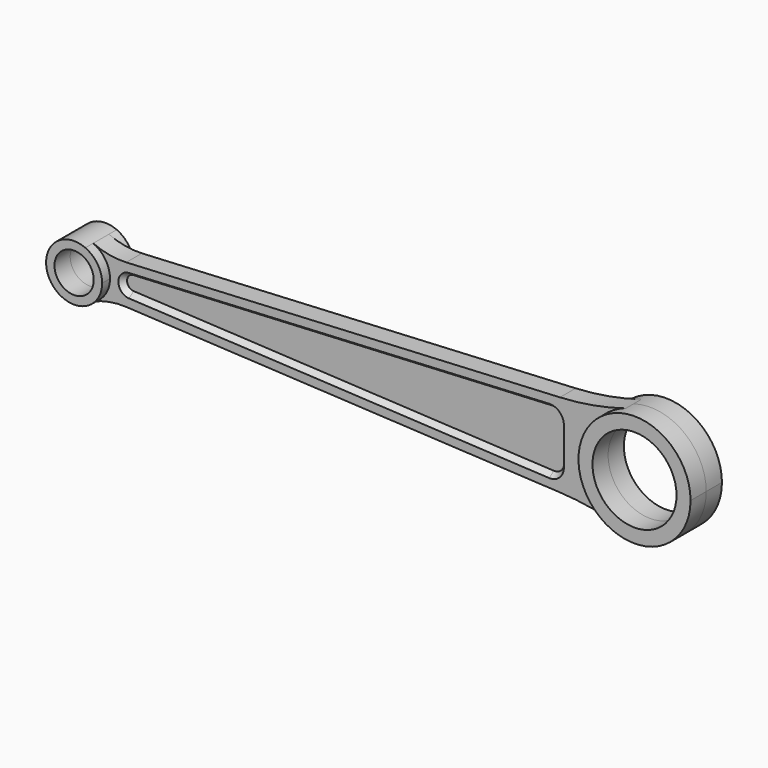
from build123d import *

# Parameters (mm, degrees)
F2_DEPTH = 3.5
F0_R     = 15
F0_R_2   = 7
F3_DEPTH = 7


# Not quite as in the source:
# - a pattern or mirror of a feature is missing from the dataset's text; its kind, count and spacing are read off the source's solid


with BuildPart() as f2:
    # F0 (on Front) → F2 (new body, symmetric)
    with BuildSketch(Plane.XZ):
        with BuildLine():
            ThreePointArc((4.0181641166, 9.157202473), (8.372026074, 5.4689285438), (10, 0))
            ThreePointArc((10, 0), (8.372026074, -5.4689285438), (4.0181641166, -9.157202473))
            ThreePointArc((4.0181641166, -9.157202473), (9.7812118117, -7.3913621026), (15.7960057944, -7))
            Line((15.7960057944, -7), (170.5928896385, -14.9325123484))
            ThreePointArc((170.5928896385, -14.9325123484), (182.467918995, -16.2860219438), (194.0827327125, -19.1046054094))
            ThreePointArc((194.0827327125, -19.1046054094), (180, 0), (194.0827327125, 19.1046054094))
            ThreePointArc((194.0827327125, 19.1046054094), (182.467918995, 16.2860219438), (170.5928896385, 14.9325123484))
            Line((170.5928896385, 14.9325123484), (15.7960057944, 7))
            ThreePointArc((15.7960057944, 7), (9.7812118117, 7.3913621026), (4.0181641166, 9.157202473))
        make_face()
    extrude(amount=F2_DEPTH, both=True)

    # F0 (on Front) → F3 (join, symmetric)
    with BuildSketch(Plane.XZ):
        with BuildLine():
            ThreePointArc((220, 0), (211.86706902, 16.0988407308), (194.0827327125, 19.1046054094))
            ThreePointArc((194.0827327125, 19.1046054094), (180, 0), (194.0827327125, -19.1046054094))
            ThreePointArc((194.0827327125, -19.1046054094), (211.86706902, -16.0988407308), (220, 0))
        make_face()
        with Locations((200, 0)):
            Circle(F0_R, mode=Mode.SUBTRACT)
        with BuildLine():
            ThreePointArc((4.0181641166, -9.157202473), (8.372026074, -5.4689285438), (10, 0))
            ThreePointArc((10, 0), (8.372026074, 5.4689285438), (4.0181641166, 9.157202473))
            ThreePointArc((4.0181641166, 9.157202473), (-10, 0), (4.0181641166, -9.157202473))
        make_face()
        Circle(F0_R_2, mode=Mode.SUBTRACT)
    extrude(amount=F3_DEPTH, both=True)

    # F5 (on offset) → F6 section 0
    with BuildSketch(Plane.XZ.offset(1.5)):
        with BuildLine():
            Line((166.8208787534, 10.1807990679), (16.8720562524, 2.496723933))
            ThreePointArc((16.8720562524, 2.496723933), (14.5, 0), (16.8720562524, -2.496723933))
            Line((16.8720562524, -2.496723933), (166.8208787534, -10.1807990679))
            ThreePointArc((166.8208787534, -10.1807990679), (169.4107131348, -9.2227980591), (170.5, -6.6853855618))
            Line((170.5, -6.6853855618), (170.5, 6.6853855618))
            ThreePointArc((170.5, 6.6853855618), (169.4107131348, 9.2227980591), (166.8208787534, 10.1807990679))
        make_face()
    # F4 (on face) → F6 section 1
    with BuildSketch(Plane.XZ.offset(3.5)):
        with BuildLine():
            Line((166.7441125049, 11.6788334277), (16.7952900039, 3.9947582928))
            ThreePointArc((16.7952900039, 3.9947582928), (13, 0), (16.7952900039, -3.9947582928))
            Line((16.7952900039, -3.9947582928), (166.7441125049, -11.6788334277))
            ThreePointArc((166.7441125049, -11.6788334277), (170.4438759069, -10.3102605579), (172, -6.6853855618))
            Line((172, -6.6853855618), (172, 6.6853855618))
            ThreePointArc((172, 6.6853855618), (170.4438759069, 10.3102605579), (166.7441125049, 11.6788334277))
        make_face()
    f6 = loft(mode=Mode.SUBTRACT)

    # F6_copies: F6 across plane
    add(f6.mirror(Plane.ZX), mode=Mode.SUBTRACT)


solid = f2.part
